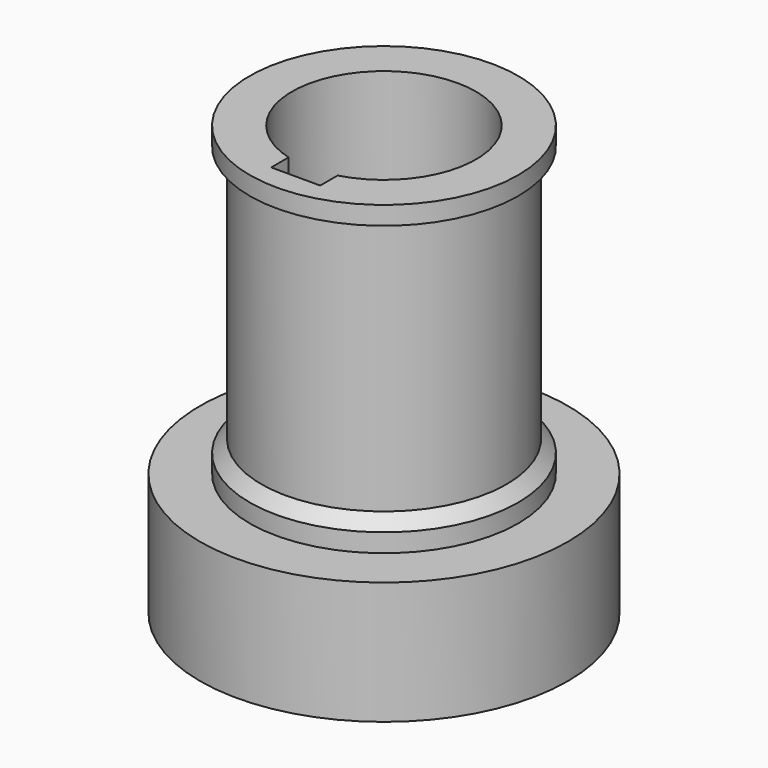
from build123d import *

# Parameters (mm, degrees)
F0_R      = 30
F1_DEPTH  = 20
F3_R      = 21.9
F4_DEPTH  = 3
F6_R      = 21.9
F7_DEPTH  = 2
F9_R      = 20
F10_DEPTH = 42
F12_R     = 21.9
F13_DEPTH = 3
F15_R     = 4
F16_DEPTH = 63.4
F18_DEPTH = 171
F19_SIZE2 = 1.99999
F19_SIZE  = 1.89999


# Not quite as in the source:
# - a fillet or chamfer is up to 0.001 mm smaller than in the source, because OpenCascade refuses the exact size


with BuildPart() as f1:
    # F0 (on Top) → F1 (new body)
    with BuildSketch(Plane.XY):
        Circle(F0_R)
    extrude(amount=F1_DEPTH)

    # F15 (on Right) → F16 (cut)
    with BuildSketch(Plane.YZ):
        with Locations((0, 10)):
            Circle(F15_R)
    extrude(amount=-F16_DEPTH, mode=Mode.SUBTRACT)


with BuildPart() as f4:
    # F3 (on offset) → F4 (new body)
    with BuildSketch(Plane.XY.offset(20)):
        Circle(F3_R)
    extrude(amount=F4_DEPTH)

    # F6 (on offset) → F7 (join)
    with BuildSketch(Plane.XY.offset(23)):
        Circle(F6_R)
    extrude(amount=F7_DEPTH)

    # F9 (on offset) → F10 (join)
    with BuildSketch(Plane.XY.offset(25)):
        Circle(F9_R)
    extrude(amount=F10_DEPTH)

    # F12 (on offset) → F13 (join)
    with BuildSketch(Plane.XY.offset(67)):
        Circle(F12_R)
    extrude(amount=F13_DEPTH)


with BuildPart() as f18_tool:
    # F17 (on offset) → F18 (new body)
    with BuildSketch(Plane.XY.offset(70)):
        with BuildLine():
            Line((4, -18), (4, -14.4568322948))
            ThreePointArc((4, -14.4568322948), (0, 15), (-4, -14.4568322948))
            Line((-4, -14.4568322948), (-4, -18))
            Line((-4, -18), (4, -18))
        make_face()
    extrude(amount=-F18_DEPTH)


with BuildPart() as f1_1:
    add(f1.part)

    # F18: cut by f18_tool
    add(f18_tool.part, mode=Mode.SUBTRACT)


with BuildPart() as f4_1:
    add(f4.part)

    # F18: cut by f18_tool
    add(f18_tool.part, mode=Mode.SUBTRACT)

    # F19 (size 1.9 and 2 in the source; OpenCascade refuses exactly that, so slightly less here)
    f19_edges = [f4_1.edges().sort_by_distance(p)[0] for p in [
        (-21.9, 0, 25),
    ]]
    f19_side = f4_1.faces().sort_by_distance((-21.280574, 0, 25))[0]
    chamfer(f19_edges, length=F19_SIZE, length2=F19_SIZE2, reference=f19_side)


solid = Compound([f1_1.part, f4_1.part])
